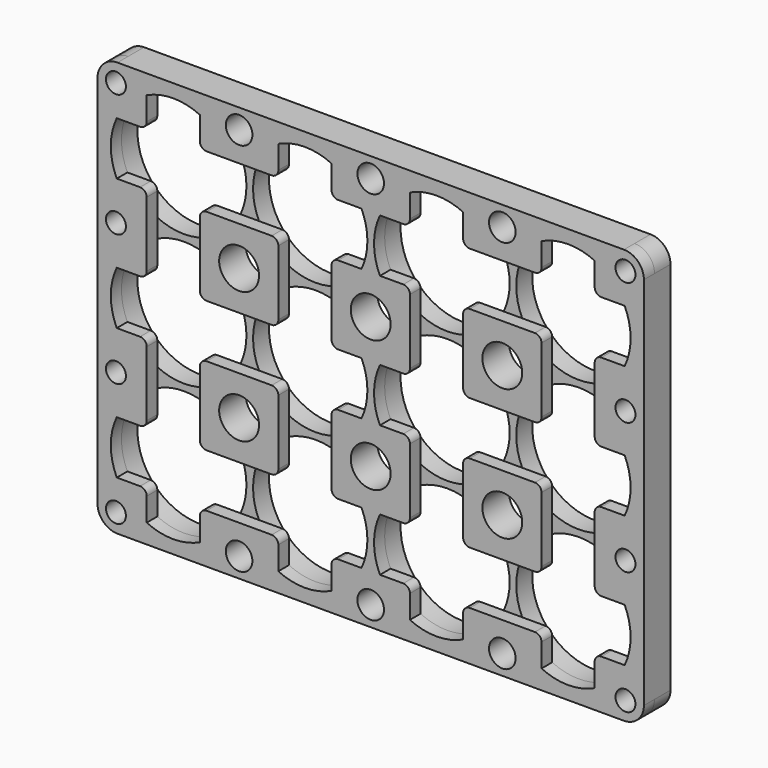
from build123d import *

# Parameters (mm, degrees)
F0_W     = 82.2
F0_H     = 62.4
F0_R     = 1.5
F0_R_2   = 9.4
F0_R_3   = 2
F0_R_4   = 3
F1_DEPTH = 3
F2_R     = 3
F3_R     = 1.5
F3_R_2   = 2
F3_R_3   = 3
F4_DEPTH = 2
F5_R     = 1


# Not quite as in the source:
# - after a boolean that leaves OpenCascade's solid faulty, fix() repairs it


with BuildPart() as f1:
    # F0 (on Front) → F1 (new body)
    with BuildSketch(Plane.XZ):
        with Locations((29.7, 19.8)):
            Rectangle(F0_W, F0_H)
        with Locations((-8.630645927, -8.630645927)):
            Circle(F0_R, mode=Mode.SUBTRACT)
        Circle(F0_R_2, mode=Mode.SUBTRACT)
        with Locations((9.9, -8.4255563615)):
            Circle(F0_R_3, mode=Mode.SUBTRACT)
        with Locations((19.8, 0)):
            Circle(F0_R_2, mode=Mode.SUBTRACT)
        with Locations((-8.630645927, 9.9)):
            Circle(F0_R, mode=Mode.SUBTRACT)
        with Locations((9.9, 9.9)):
            Circle(F0_R_4, mode=Mode.SUBTRACT)
        with Locations((29.7, -8.4255563615)):
            Circle(F0_R_3, mode=Mode.SUBTRACT)
        with Locations((49.5, -8.4255563615)):
            Circle(F0_R_3, mode=Mode.SUBTRACT)
        with Locations((39.6, 0)):
            Circle(F0_R_2, mode=Mode.SUBTRACT)
        with Locations((68.030645927, -8.630645927)):
            Circle(F0_R, mode=Mode.SUBTRACT)
        with Locations((59.4, 0)):
            Circle(F0_R_2, mode=Mode.SUBTRACT)
        with Locations((29.7, 9.9)):
            Circle(F0_R_4, mode=Mode.SUBTRACT)
        with Locations((49.5, 9.9)):
            Circle(F0_R_4, mode=Mode.SUBTRACT)
        with Locations((68.030645927, 9.9)):
            Circle(F0_R, mode=Mode.SUBTRACT)
        with Locations((0, 19.8)):
            Circle(F0_R_2, mode=Mode.SUBTRACT)
        with Locations((-8.630645927, 29.7)):
            Circle(F0_R, mode=Mode.SUBTRACT)
        with Locations((19.8, 19.8)):
            Circle(F0_R_2, mode=Mode.SUBTRACT)
        with Locations((9.9, 29.7)):
            Circle(F0_R_4, mode=Mode.SUBTRACT)
        with Locations((0, 39.6)):
            Circle(F0_R_2, mode=Mode.SUBTRACT)
        with Locations((-8.630645927, 48.230645927)):
            Circle(F0_R, mode=Mode.SUBTRACT)
        with Locations((19.8, 39.6)):
            Circle(F0_R_2, mode=Mode.SUBTRACT)
        with Locations((9.9, 48.0255563615)):
            Circle(F0_R_3, mode=Mode.SUBTRACT)
        with Locations((39.6, 19.8)):
            Circle(F0_R_2, mode=Mode.SUBTRACT)
        with Locations((29.7, 29.7)):
            Circle(F0_R_4, mode=Mode.SUBTRACT)
        with Locations((49.5, 29.7)):
            Circle(F0_R_4, mode=Mode.SUBTRACT)
        with Locations((59.4, 19.8)):
            Circle(F0_R_2, mode=Mode.SUBTRACT)
        with Locations((68.030645927, 29.7)):
            Circle(F0_R, mode=Mode.SUBTRACT)
        with Locations((39.6, 39.6)):
            Circle(F0_R_2, mode=Mode.SUBTRACT)
        with Locations((29.7, 48.0255563615)):
            Circle(F0_R_3, mode=Mode.SUBTRACT)
        with Locations((49.5, 48.0255563615)):
            Circle(F0_R_3, mode=Mode.SUBTRACT)
        with Locations((59.4, 39.6)):
            Circle(F0_R_2, mode=Mode.SUBTRACT)
        with Locations((68.030645927, 48.230645927)):
            Circle(F0_R, mode=Mode.SUBTRACT)
    extrude(amount=F1_DEPTH)

    # F2
    f2_edges = [f1.edges().sort_by_distance(p)[0] for p in [
        (70.8, -1.5, 51),
        (-11.4, -1.5, 51),
        (-11.4, -1.5, -11.4),
        (70.8, -1.5, -11.4),
    ]]
    fillet(f2_edges, radius=F2_R)

    # F3 (on face) → F4 (join)
    with BuildSketch(Plane.XZ.offset(3)):
        with BuildLine():
            ThreePointArc((70.8, 48), (69.9213203436, 50.1213203436), (67.8, 51))
            Line((67.8, 51), (63.4, 51))
            Line((63.4, 51), (63.4, 48.1064681273))
            ThreePointArc((63.4, 48.1064681273), (66.0468037432, 46.2468037432), (67.9064681273, 43.6))
            Line((67.9064681273, 43.6), (70.8, 43.6))
            Line((70.8, 43.6), (70.8, 48))
        make_face()
        with Locations((68.030645927, 48.230645927)):
            Circle(F3_R, mode=Mode.SUBTRACT)
        with BuildLine():
            Line((63.4, 48.1064681273), (63.4, 51))
            Line((63.4, 51), (55.4, 51))
            Line((55.4, 51), (55.4, 48.1064681273))
            ThreePointArc((55.4, 48.1064681273), (59.4, 49), (63.4, 48.1064681273))
        make_face()
        with BuildLine():
            Line((55.4, 48.1064681273), (55.4, 51))
            Line((55.4, 51), (43.6, 51))
            Line((43.6, 51), (43.6, 48.1064681273))
            ThreePointArc((43.6, 48.1064681273), (46.2468037432, 46.2468037432), (48.1064681273, 43.6))
            Line((48.1064681273, 43.6), (50.8935318727, 43.6))
            ThreePointArc((50.8935318727, 43.6), (52.7531962568, 46.2468037432), (55.4, 48.1064681273))
        make_face()
        with Locations((49.5, 48.0255563615)):
            Circle(F3_R_2, mode=Mode.SUBTRACT)
        with BuildLine():
            ThreePointArc((67.9064681273, 43.6), (66.0468037432, 46.2468037432), (63.4, 48.1064681273))
            Line((63.4, 48.1064681273), (63.4, 43.6))
            Line((63.4, 43.6), (67.9064681273, 43.6))
        make_face()
        with BuildLine():
            Line((70.8, 39.6), (70.8, 43.6))
            Line((70.8, 43.6), (67.9064681273, 43.6))
            ThreePointArc((67.9064681273, 43.6), (68.5738977648, 41.6492925125), (68.8, 39.6))
            ThreePointArc((68.8, 39.6), (68.5738977648, 37.5507074875), (67.9064681273, 35.6))
            Line((67.9064681273, 35.6), (70.8, 35.6))
            Line((70.8, 35.6), (70.8, 39.6))
        make_face()
        with BuildLine():
            Line((43.6, 48.1064681273), (43.6, 51))
            Line((43.6, 51), (35.6, 51))
            Line((35.6, 51), (35.6, 48.1064681273))
            ThreePointArc((35.6, 48.1064681273), (39.6, 49), (43.6, 48.1064681273))
        make_face()
        with BuildLine():
            Line((55.4, 43.6), (55.4, 48.1064681273))
            ThreePointArc((55.4, 48.1064681273), (52.7531962568, 46.2468037432), (50.8935318727, 43.6))
            Line((50.8935318727, 43.6), (55.4, 43.6))
        make_face()
        with BuildLine():
            Line((35.6, 48.1064681273), (35.6, 51))
            Line((35.6, 51), (23.8, 51))
            Line((23.8, 51), (23.8, 48.1064681273))
            ThreePointArc((23.8, 48.1064681273), (26.4468037432, 46.2468037432), (28.3064681273, 43.6))
            Line((28.3064681273, 43.6), (31.0935318727, 43.6))
            ThreePointArc((31.0935318727, 43.6), (32.9531962568, 46.2468037432), (35.6, 48.1064681273))
        make_face()
        with Locations((29.7, 48.0255563615)):
            Circle(F3_R_2, mode=Mode.SUBTRACT)
        with BuildLine():
            ThreePointArc((48.1064681273, 43.6), (46.2468037432, 46.2468037432), (43.6, 48.1064681273))
            Line((43.6, 48.1064681273), (43.6, 43.6))
            Line((43.6, 43.6), (48.1064681273, 43.6))
        make_face()
        with BuildLine():
            Line((70.8, 23.8), (70.8, 35.6))
            Line((70.8, 35.6), (67.9064681273, 35.6))
            ThreePointArc((67.9064681273, 35.6), (66.0468037432, 32.9531962568), (63.4, 31.0935318727))
            Line((63.4, 31.0935318727), (63.4, 28.3064681273))
            ThreePointArc((63.4, 28.3064681273), (66.0468037432, 26.4468037432), (67.9064681273, 23.8))
            Line((67.9064681273, 23.8), (70.8, 23.8))
        make_face()
        with Locations((68.030645927, 29.7)):
            Circle(F3_R, mode=Mode.SUBTRACT)
        with BuildLine():
            Line((23.8, 48.1064681273), (23.8, 51))
            Line((23.8, 51), (15.8, 51))
            Line((15.8, 51), (15.8, 48.1064681273))
            ThreePointArc((15.8, 48.1064681273), (19.8, 49), (23.8, 48.1064681273))
        make_face()
        with BuildLine():
            Line((35.6, 43.6), (35.6, 48.1064681273))
            ThreePointArc((35.6, 48.1064681273), (32.9531962568, 46.2468037432), (31.0935318727, 43.6))
            Line((31.0935318727, 43.6), (35.6, 43.6))
        make_face()
        with BuildLine():
            Line((55.4, 35.6), (50.8935318727, 35.6))
            ThreePointArc((50.8935318727, 35.6), (52.7531962568, 32.9531962568), (55.4, 31.0935318727))
            Line((55.4, 31.0935318727), (55.4, 35.6))
        make_face()
        with BuildLine():
            ThreePointArc((55.4, 31.0935318727), (52.7531962568, 32.9531962568), (50.8935318727, 35.6))
            Line((50.8935318727, 35.6), (48.1064681273, 35.6))
            ThreePointArc((48.1064681273, 35.6), (46.2468037432, 32.9531962568), (43.6, 31.0935318727))
            Line((43.6, 31.0935318727), (43.6, 28.3064681273))
            ThreePointArc((43.6, 28.3064681273), (46.2468037432, 26.4468037432), (48.1064681273, 23.8))
            Line((48.1064681273, 23.8), (50.8935318727, 23.8))
            ThreePointArc((50.8935318727, 23.8), (52.7531962568, 26.4468037432), (55.4, 28.3064681273))
            Line((55.4, 28.3064681273), (55.4, 31.0935318727))
        make_face()
        with Locations((49.5, 29.7)):
            Circle(F3_R_3, mode=Mode.SUBTRACT)
        with BuildLine():
            ThreePointArc((63.4, 31.0935318727), (66.0468037432, 32.9531962568), (67.9064681273, 35.6))
            Line((67.9064681273, 35.6), (63.4, 35.6))
            Line((63.4, 35.6), (63.4, 31.0935318727))
        make_face()
        with BuildLine():
            Line((70.8, 15.8), (70.8, 23.8))
            Line((70.8, 23.8), (67.9064681273, 23.8))
            ThreePointArc((67.9064681273, 23.8), (68.5738977648, 21.8492925125), (68.8, 19.8))
            ThreePointArc((68.8, 19.8), (68.5738977648, 17.7507074875), (67.9064681273, 15.8))
            Line((67.9064681273, 15.8), (70.8, 15.8))
        make_face()
        with BuildLine():
            Line((15.8, 48.1064681273), (15.8, 51))
            Line((15.8, 51), (4, 51))
            Line((4, 51), (4, 48.1064681273))
            ThreePointArc((4, 48.1064681273), (6.6468037432, 46.2468037432), (8.5064681273, 43.6))
            Line((8.5064681273, 43.6), (11.2935318727, 43.6))
            ThreePointArc((11.2935318727, 43.6), (13.1531962568, 46.2468037432), (15.8, 48.1064681273))
        make_face()
        with Locations((9.9, 48.0255563615)):
            Circle(F3_R_2, mode=Mode.SUBTRACT)
        with BuildLine():
            ThreePointArc((28.3064681273, 43.6), (26.4468037432, 46.2468037432), (23.8, 48.1064681273))
            Line((23.8, 48.1064681273), (23.8, 43.6))
            Line((23.8, 43.6), (28.3064681273, 43.6))
        make_face()
        with BuildLine():
            ThreePointArc((31.0935318727, 35.6), (30.2, 39.6), (31.0935318727, 43.6))
            Line((31.0935318727, 43.6), (28.3064681273, 43.6))
            ThreePointArc((28.3064681273, 43.6), (28.9738977648, 41.6492925125), (29.2, 39.6))
            ThreePointArc((29.2, 39.6), (28.9738977648, 37.5507074875), (28.3064681273, 35.6))
            Line((28.3064681273, 35.6), (31.0935318727, 35.6))
        make_face()
        with BuildLine():
            ThreePointArc((43.6, 31.0935318727), (46.2468037432, 32.9531962568), (48.1064681273, 35.6))
            Line((48.1064681273, 35.6), (43.6, 35.6))
            Line((43.6, 35.6), (43.6, 31.0935318727))
        make_face()
        with BuildLine():
            Line((70.8, 4), (70.8, 15.8))
            Line((70.8, 15.8), (67.9064681273, 15.8))
            ThreePointArc((67.9064681273, 15.8), (66.0468037432, 13.1531962568), (63.4, 11.2935318727))
            Line((63.4, 11.2935318727), (63.4, 8.5064681273))
            ThreePointArc((63.4, 8.5064681273), (66.0468037432, 6.6468037432), (67.9064681273, 4))
            Line((67.9064681273, 4), (70.8, 4))
        make_face()
        with Locations((68.030645927, 9.9)):
            Circle(F3_R, mode=Mode.SUBTRACT)
        with BuildLine():
            Line((63.4, 23.8), (67.9064681273, 23.8))
            ThreePointArc((67.9064681273, 23.8), (66.0468037432, 26.4468037432), (63.4, 28.3064681273))
            Line((63.4, 28.3064681273), (63.4, 23.8))
        make_face()
        with BuildLine():
            Line((4, 48.1064681273), (4, 51))
            Line((4, 51), (-4, 51))
            Line((-4, 51), (-4, 48.1064681273))
            ThreePointArc((-4, 48.1064681273), (0, 49), (4, 48.1064681273))
        make_face()
        with BuildLine():
            Line((15.8, 43.6), (15.8, 48.1064681273))
            ThreePointArc((15.8, 48.1064681273), (13.1531962568, 46.2468037432), (11.2935318727, 43.6))
            Line((11.2935318727, 43.6), (15.8, 43.6))
        make_face()
        with BuildLine():
            Line((35.6, 35.6), (31.0935318727, 35.6))
            ThreePointArc((31.0935318727, 35.6), (32.9531962568, 32.9531962568), (35.6, 31.0935318727))
            Line((35.6, 31.0935318727), (35.6, 35.6))
        make_face()
        with BuildLine():
            ThreePointArc((35.6, 31.0935318727), (32.9531962568, 32.9531962568), (31.0935318727, 35.6))
            Line((31.0935318727, 35.6), (28.3064681273, 35.6))
            ThreePointArc((28.3064681273, 35.6), (26.4468037432, 32.9531962568), (23.8, 31.0935318727))
            Line((23.8, 31.0935318727), (23.8, 28.3064681273))
            ThreePointArc((23.8, 28.3064681273), (26.4468037432, 26.4468037432), (28.3064681273, 23.8))
            Line((28.3064681273, 23.8), (31.0935318727, 23.8))
            ThreePointArc((31.0935318727, 23.8), (32.9531962568, 26.4468037432), (35.6, 28.3064681273))
            Line((35.6, 28.3064681273), (35.6, 31.0935318727))
        make_face()
        with Locations((29.7, 29.7)):
            Circle(F3_R_3, mode=Mode.SUBTRACT)
        with BuildLine():
            Line((55.4, 23.8), (55.4, 28.3064681273))
            ThreePointArc((55.4, 28.3064681273), (52.7531962568, 26.4468037432), (50.8935318727, 23.8))
            Line((50.8935318727, 23.8), (55.4, 23.8))
        make_face()
        with BuildLine():
            Line((70.8, -4), (70.8, 4))
            Line((70.8, 4), (67.9064681273, 4))
            ThreePointArc((67.9064681273, 4), (68.5738977648, 2.0492925125), (68.8, 0))
            ThreePointArc((68.8, 0), (68.5738977648, -2.0492925125), (67.9064681273, -4))
            Line((67.9064681273, -4), (70.8, -4))
        make_face()
        with BuildLine():
            ThreePointArc((63.4, 11.2935318727), (66.0468037432, 13.1531962568), (67.9064681273, 15.8))
            Line((67.9064681273, 15.8), (63.4, 15.8))
            Line((63.4, 15.8), (63.4, 11.2935318727))
        make_face()
        with BuildLine():
            Line((-4, 48.1064681273), (-4, 51))
            Line((-4, 51), (-8.4, 51))
            ThreePointArc((-8.4, 51), (-10.5213203436, 50.1213203436), (-11.4, 48))
            Line((-11.4, 48), (-11.4, 43.6))
            Line((-11.4, 43.6), (-8.5064681273, 43.6))
            ThreePointArc((-8.5064681273, 43.6), (-6.6468037432, 46.2468037432), (-4, 48.1064681273))
        make_face()
        with Locations((-8.630645927, 48.230645927)):
            Circle(F3_R, mode=Mode.SUBTRACT)
        with BuildLine():
            ThreePointArc((8.5064681273, 43.6), (6.6468037432, 46.2468037432), (4, 48.1064681273))
            Line((4, 48.1064681273), (4, 43.6))
            Line((4, 43.6), (8.5064681273, 43.6))
        make_face()
        with BuildLine():
            ThreePointArc((23.8, 31.0935318727), (26.4468037432, 32.9531962568), (28.3064681273, 35.6))
            Line((28.3064681273, 35.6), (23.8, 35.6))
            Line((23.8, 35.6), (23.8, 31.0935318727))
        make_face()
        with BuildLine():
            ThreePointArc((48.1064681273, 23.8), (46.2468037432, 26.4468037432), (43.6, 28.3064681273))
            Line((43.6, 28.3064681273), (43.6, 23.8))
            Line((43.6, 23.8), (48.1064681273, 23.8))
        make_face()
        with BuildLine():
            Line((70.8, -8.4), (70.8, -4))
            Line((70.8, -4), (67.9064681273, -4))
            ThreePointArc((67.9064681273, -4), (66.0468037432, -6.6468037432), (63.4, -8.5064681273))
            Line((63.4, -8.5064681273), (63.4, -11.4))
            Line((63.4, -11.4), (67.8, -11.4))
            ThreePointArc((67.8, -11.4), (69.9213203436, -10.5213203436), (70.8, -8.4))
        make_face()
        with Locations((68.030645927, -8.630645927)):
            Circle(F3_R, mode=Mode.SUBTRACT)
        with BuildLine():
            Line((63.4, 4), (67.9064681273, 4))
            ThreePointArc((67.9064681273, 4), (66.0468037432, 6.6468037432), (63.4, 8.5064681273))
            Line((63.4, 8.5064681273), (63.4, 4))
        make_face()
        with BuildLine():
            Line((-4, 43.6), (-4, 48.1064681273))
            ThreePointArc((-4, 48.1064681273), (-6.6468037432, 46.2468037432), (-8.5064681273, 43.6))
            Line((-8.5064681273, 43.6), (-4, 43.6))
        make_face()
        with BuildLine():
            Line((15.8, 35.6), (11.2935318727, 35.6))
            ThreePointArc((11.2935318727, 35.6), (13.1531962568, 32.9531962568), (15.8, 31.0935318727))
            Line((15.8, 31.0935318727), (15.8, 35.6))
        make_face()
        with BuildLine():
            ThreePointArc((15.8, 31.0935318727), (13.1531962568, 32.9531962568), (11.2935318727, 35.6))
            Line((11.2935318727, 35.6), (8.5064681273, 35.6))
            ThreePointArc((8.5064681273, 35.6), (6.6468037432, 32.9531962568), (4, 31.0935318727))
            Line((4, 31.0935318727), (4, 28.3064681273))
            ThreePointArc((4, 28.3064681273), (6.6468037432, 26.4468037432), (8.5064681273, 23.8))
            Line((8.5064681273, 23.8), (11.2935318727, 23.8))
            ThreePointArc((11.2935318727, 23.8), (13.1531962568, 26.4468037432), (15.8, 28.3064681273))
            Line((15.8, 28.3064681273), (15.8, 31.0935318727))
        make_face()
        with Locations((9.9, 29.7)):
            Circle(F3_R_3, mode=Mode.SUBTRACT)
        with BuildLine():
            Line((35.6, 23.8), (35.6, 28.3064681273))
            ThreePointArc((35.6, 28.3064681273), (32.9531962568, 26.4468037432), (31.0935318727, 23.8))
            Line((31.0935318727, 23.8), (35.6, 23.8))
        make_face()
        with BuildLine():
            Line((55.4, 15.8), (50.8935318727, 15.8))
            ThreePointArc((50.8935318727, 15.8), (52.7531962568, 13.1531962568), (55.4, 11.2935318727))
            Line((55.4, 11.2935318727), (55.4, 15.8))
        make_face()
        with BuildLine():
            ThreePointArc((55.4, 11.2935318727), (52.7531962568, 13.1531962568), (50.8935318727, 15.8))
            Line((50.8935318727, 15.8), (48.1064681273, 15.8))
            ThreePointArc((48.1064681273, 15.8), (46.2468037432, 13.1531962568), (43.6, 11.2935318727))
            Line((43.6, 11.2935318727), (43.6, 8.5064681273))
            ThreePointArc((43.6, 8.5064681273), (46.2468037432, 6.6468037432), (48.1064681273, 4))
            Line((48.1064681273, 4), (50.8935318727, 4))
            ThreePointArc((50.8935318727, 4), (52.7531962568, 6.6468037432), (55.4, 8.5064681273))
            Line((55.4, 8.5064681273), (55.4, 11.2935318727))
        make_face()
        with Locations((49.5, 9.9)):
            Circle(F3_R_3, mode=Mode.SUBTRACT)
        with BuildLine():
            ThreePointArc((63.4, -8.5064681273), (66.0468037432, -6.6468037432), (67.9064681273, -4))
            Line((67.9064681273, -4), (63.4, -4))
            Line((63.4, -4), (63.4, -8.5064681273))
        make_face()
        with BuildLine():
            ThreePointArc((-8.5064681273, 35.6), (-9.4, 39.6), (-8.5064681273, 43.6))
            Line((-8.5064681273, 43.6), (-11.4, 43.6))
            Line((-11.4, 43.6), (-11.4, 39.6))
            Line((-11.4, 39.6), (-11.4, 35.6))
            Line((-11.4, 35.6), (-8.5064681273, 35.6))
        make_face()
        with BuildLine():
            ThreePointArc((4, 31.0935318727), (6.6468037432, 32.9531962568), (8.5064681273, 35.6))
            Line((8.5064681273, 35.6), (4, 35.6))
            Line((4, 35.6), (4, 31.0935318727))
        make_face()
        with BuildLine():
            ThreePointArc((31.0935318727, 15.8), (30.2, 19.8), (31.0935318727, 23.8))
            Line((31.0935318727, 23.8), (28.3064681273, 23.8))
            ThreePointArc((28.3064681273, 23.8), (28.9738977648, 21.8492925125), (29.2, 19.8))
            ThreePointArc((29.2, 19.8), (28.9738977648, 17.7507074875), (28.3064681273, 15.8))
            Line((28.3064681273, 15.8), (31.0935318727, 15.8))
        make_face()
        with BuildLine():
            ThreePointArc((28.3064681273, 23.8), (26.4468037432, 26.4468037432), (23.8, 28.3064681273))
            Line((23.8, 28.3064681273), (23.8, 23.8))
            Line((23.8, 23.8), (28.3064681273, 23.8))
        make_face()
        with BuildLine():
            ThreePointArc((43.6, 11.2935318727), (46.2468037432, 13.1531962568), (48.1064681273, 15.8))
            Line((48.1064681273, 15.8), (43.6, 15.8))
            Line((43.6, 15.8), (43.6, 11.2935318727))
        make_face()
        with BuildLine():
            Line((63.4, -11.4), (63.4, -8.5064681273))
            ThreePointArc((63.4, -8.5064681273), (59.4, -9.4), (55.4, -8.5064681273))
            Line((55.4, -8.5064681273), (55.4, -11.4))
            Line((55.4, -11.4), (63.4, -11.4))
        make_face()
        with BuildLine():
            Line((55.4, 4), (55.4, 8.5064681273))
            ThreePointArc((55.4, 8.5064681273), (52.7531962568, 6.6468037432), (50.8935318727, 4))
            Line((50.8935318727, 4), (55.4, 4))
        make_face()
        with BuildLine():
            ThreePointArc((-4, 31.0935318727), (-6.6468037432, 32.9531962568), (-8.5064681273, 35.6))
            Line((-8.5064681273, 35.6), (-11.4, 35.6))
            Line((-11.4, 35.6), (-11.4, 23.8))
            Line((-11.4, 23.8), (-8.5064681273, 23.8))
            ThreePointArc((-8.5064681273, 23.8), (-6.6468037432, 26.4468037432), (-4, 28.3064681273))
            Line((-4, 28.3064681273), (-4, 31.0935318727))
        make_face()
        with Locations((-8.630645927, 29.7)):
            Circle(F3_R, mode=Mode.SUBTRACT)
        with BuildLine():
            Line((-4, 35.6), (-8.5064681273, 35.6))
            ThreePointArc((-8.5064681273, 35.6), (-6.6468037432, 32.9531962568), (-4, 31.0935318727))
            Line((-4, 31.0935318727), (-4, 35.6))
        make_face()
        with BuildLine():
            Line((15.8, 23.8), (15.8, 28.3064681273))
            ThreePointArc((15.8, 28.3064681273), (13.1531962568, 26.4468037432), (11.2935318727, 23.8))
            Line((11.2935318727, 23.8), (15.8, 23.8))
        make_face()
        with BuildLine():
            Line((35.6, 15.8), (31.0935318727, 15.8))
            ThreePointArc((31.0935318727, 15.8), (32.9531962568, 13.1531962568), (35.6, 11.2935318727))
            Line((35.6, 11.2935318727), (35.6, 15.8))
        make_face()
        with BuildLine():
            ThreePointArc((35.6, 11.2935318727), (32.9531962568, 13.1531962568), (31.0935318727, 15.8))
            Line((31.0935318727, 15.8), (28.3064681273, 15.8))
            ThreePointArc((28.3064681273, 15.8), (26.4468037432, 13.1531962568), (23.8, 11.2935318727))
            Line((23.8, 11.2935318727), (23.8, 8.5064681273))
            ThreePointArc((23.8, 8.5064681273), (26.4468037432, 6.6468037432), (28.3064681273, 4))
            Line((28.3064681273, 4), (31.0935318727, 4))
            ThreePointArc((31.0935318727, 4), (32.9531962568, 6.6468037432), (35.6, 8.5064681273))
            Line((35.6, 8.5064681273), (35.6, 11.2935318727))
        make_face()
        with Locations((29.7, 9.9)):
            Circle(F3_R_3, mode=Mode.SUBTRACT)
        with BuildLine():
            Line((55.4, -11.4), (55.4, -8.5064681273))
            ThreePointArc((55.4, -8.5064681273), (52.7531962568, -6.6468037432), (50.8935318727, -4))
            Line((50.8935318727, -4), (48.1064681273, -4))
            ThreePointArc((48.1064681273, -4), (46.2468037432, -6.6468037432), (43.6, -8.5064681273))
            Line((43.6, -8.5064681273), (43.6, -11.4))
            Line((43.6, -11.4), (55.4, -11.4))
        make_face()
        with Locations((49.5, -8.4255563615)):
            Circle(F3_R_2, mode=Mode.SUBTRACT)
        with BuildLine():
            ThreePointArc((50.8935318727, -4), (52.7531962568, -6.6468037432), (55.4, -8.5064681273))
            Line((55.4, -8.5064681273), (55.4, -4))
            Line((55.4, -4), (50.8935318727, -4))
        make_face()
        with BuildLine():
            ThreePointArc((8.5064681273, 23.8), (6.6468037432, 26.4468037432), (4, 28.3064681273))
            Line((4, 28.3064681273), (4, 23.8))
            Line((4, 23.8), (8.5064681273, 23.8))
        make_face()
        with BuildLine():
            ThreePointArc((23.8, 11.2935318727), (26.4468037432, 13.1531962568), (28.3064681273, 15.8))
            Line((28.3064681273, 15.8), (23.8, 15.8))
            Line((23.8, 15.8), (23.8, 11.2935318727))
        make_face()
        with BuildLine():
            ThreePointArc((48.1064681273, 4), (46.2468037432, 6.6468037432), (43.6, 8.5064681273))
            Line((43.6, 8.5064681273), (43.6, 4))
            Line((43.6, 4), (48.1064681273, 4))
        make_face()
        with BuildLine():
            Line((-8.5064681273, 23.8), (-11.4, 23.8))
            Line((-11.4, 23.8), (-11.4, 15.8))
            Line((-11.4, 15.8), (-8.5064681273, 15.8))
            ThreePointArc((-8.5064681273, 15.8), (-9.4, 19.8), (-8.5064681273, 23.8))
        make_face()
        with BuildLine():
            Line((-4, 23.8), (-4, 28.3064681273))
            ThreePointArc((-4, 28.3064681273), (-6.6468037432, 26.4468037432), (-8.5064681273, 23.8))
            Line((-8.5064681273, 23.8), (-4, 23.8))
        make_face()
        with BuildLine():
            Line((15.8, 15.8), (11.2935318727, 15.8))
            ThreePointArc((11.2935318727, 15.8), (13.1531962568, 13.1531962568), (15.8, 11.2935318727))
            Line((15.8, 11.2935318727), (15.8, 15.8))
        make_face()
        with BuildLine():
            ThreePointArc((15.8, 11.2935318727), (13.1531962568, 13.1531962568), (11.2935318727, 15.8))
            Line((11.2935318727, 15.8), (8.5064681273, 15.8))
            ThreePointArc((8.5064681273, 15.8), (6.6468037432, 13.1531962568), (4, 11.2935318727))
            Line((4, 11.2935318727), (4, 8.5064681273))
            ThreePointArc((4, 8.5064681273), (6.6468037432, 6.6468037432), (8.5064681273, 4))
            Line((8.5064681273, 4), (11.2935318727, 4))
            ThreePointArc((11.2935318727, 4), (13.1531962568, 6.6468037432), (15.8, 8.5064681273))
            Line((15.8, 8.5064681273), (15.8, 11.2935318727))
        make_face()
        with Locations((9.9, 9.9)):
            Circle(F3_R_3, mode=Mode.SUBTRACT)
        with BuildLine():
            Line((35.6, 4), (35.6, 8.5064681273))
            ThreePointArc((35.6, 8.5064681273), (32.9531962568, 6.6468037432), (31.0935318727, 4))
            Line((31.0935318727, 4), (35.6, 4))
        make_face()
        with BuildLine():
            Line((35.6, -11.4), (43.6, -11.4))
            Line((43.6, -11.4), (43.6, -8.5064681273))
            ThreePointArc((43.6, -8.5064681273), (39.6, -9.4), (35.6, -8.5064681273))
            Line((35.6, -8.5064681273), (35.6, -11.4))
        make_face()
        with BuildLine():
            ThreePointArc((43.6, -8.5064681273), (46.2468037432, -6.6468037432), (48.1064681273, -4))
            Line((48.1064681273, -4), (43.6, -4))
            Line((43.6, -4), (43.6, -8.5064681273))
        make_face()
        with BuildLine():
            Line((-8.5064681273, 15.8), (-11.4, 15.8))
            Line((-11.4, 15.8), (-11.4, 4))
            Line((-11.4, 4), (-8.5064681273, 4))
            ThreePointArc((-8.5064681273, 4), (-6.6468037432, 6.6468037432), (-4, 8.5064681273))
            Line((-4, 8.5064681273), (-4, 11.2935318727))
            ThreePointArc((-4, 11.2935318727), (-6.6468037432, 13.1531962568), (-8.5064681273, 15.8))
        make_face()
        with Locations((-8.630645927, 9.9)):
            Circle(F3_R, mode=Mode.SUBTRACT)
        with BuildLine():
            ThreePointArc((4, 11.2935318727), (6.6468037432, 13.1531962568), (8.5064681273, 15.8))
            Line((8.5064681273, 15.8), (4, 15.8))
            Line((4, 15.8), (4, 11.2935318727))
        make_face()
        with BuildLine():
            ThreePointArc((31.0935318727, -4), (30.2, 0), (31.0935318727, 4))
            Line((31.0935318727, 4), (28.3064681273, 4))
            ThreePointArc((28.3064681273, 4), (28.9738977648, 2.0492925125), (29.2, 0))
            ThreePointArc((29.2, 0), (28.9738977648, -2.0492925125), (28.3064681273, -4))
            Line((28.3064681273, -4), (31.0935318727, -4))
        make_face()
        with BuildLine():
            ThreePointArc((28.3064681273, 4), (26.4468037432, 6.6468037432), (23.8, 8.5064681273))
            Line((23.8, 8.5064681273), (23.8, 4))
            Line((23.8, 4), (28.3064681273, 4))
        make_face()
        with BuildLine():
            Line((23.8, -11.4), (35.6, -11.4))
            Line((35.6, -11.4), (35.6, -8.5064681273))
            ThreePointArc((35.6, -8.5064681273), (32.9531962568, -6.6468037432), (31.0935318727, -4))
            Line((31.0935318727, -4), (28.3064681273, -4))
            ThreePointArc((28.3064681273, -4), (26.4468037432, -6.6468037432), (23.8, -8.5064681273))
            Line((23.8, -8.5064681273), (23.8, -11.4))
        make_face()
        with Locations((29.7, -8.4255563615)):
            Circle(F3_R_2, mode=Mode.SUBTRACT)
        with BuildLine():
            Line((-8.5064681273, 4), (-11.4, 4))
            Line((-11.4, 4), (-11.4, -4))
            Line((-11.4, -4), (-8.5064681273, -4))
            ThreePointArc((-8.5064681273, -4), (-9.4, 0), (-8.5064681273, 4))
        make_face()
        with BuildLine():
            Line((-4, 15.8), (-8.5064681273, 15.8))
            ThreePointArc((-8.5064681273, 15.8), (-6.6468037432, 13.1531962568), (-4, 11.2935318727))
            Line((-4, 11.2935318727), (-4, 15.8))
        make_face()
        with BuildLine():
            Line((15.8, 4), (15.8, 8.5064681273))
            ThreePointArc((15.8, 8.5064681273), (13.1531962568, 6.6468037432), (11.2935318727, 4))
            Line((11.2935318727, 4), (15.8, 4))
        make_face()
        with BuildLine():
            Line((35.6, -4), (31.0935318727, -4))
            ThreePointArc((31.0935318727, -4), (32.9531962568, -6.6468037432), (35.6, -8.5064681273))
            Line((35.6, -8.5064681273), (35.6, -4))
        make_face()
        with BuildLine():
            Line((15.8, -11.4), (23.8, -11.4))
            Line((23.8, -11.4), (23.8, -8.5064681273))
            ThreePointArc((23.8, -8.5064681273), (19.8, -9.4), (15.8, -8.5064681273))
            Line((15.8, -8.5064681273), (15.8, -11.4))
        make_face()
        with BuildLine():
            Line((-8.5064681273, -4), (-11.4, -4))
            Line((-11.4, -4), (-11.4, -8.4))
            ThreePointArc((-11.4, -8.4), (-10.5213203436, -10.5213203436), (-8.4, -11.4))
            Line((-8.4, -11.4), (-4, -11.4))
            Line((-4, -11.4), (-4, -8.5064681273))
            ThreePointArc((-4, -8.5064681273), (-6.6468037432, -6.6468037432), (-8.5064681273, -4))
        make_face()
        with Locations((-8.630645927, -8.630645927)):
            Circle(F3_R, mode=Mode.SUBTRACT)
        with BuildLine():
            ThreePointArc((-4, 8.5064681273), (-6.6468037432, 6.6468037432), (-8.5064681273, 4))
            Line((-8.5064681273, 4), (-4, 4))
            Line((-4, 4), (-4, 8.5064681273))
        make_face()
        with BuildLine():
            ThreePointArc((8.5064681273, 4), (6.6468037432, 6.6468037432), (4, 8.5064681273))
            Line((4, 8.5064681273), (4, 4))
            Line((4, 4), (8.5064681273, 4))
        make_face()
        with BuildLine():
            ThreePointArc((23.8, -8.5064681273), (26.4468037432, -6.6468037432), (28.3064681273, -4))
            Line((28.3064681273, -4), (23.8, -4))
            Line((23.8, -4), (23.8, -8.5064681273))
        make_face()
        with BuildLine():
            Line((4, -11.4), (15.8, -11.4))
            Line((15.8, -11.4), (15.8, -8.5064681273))
            ThreePointArc((15.8, -8.5064681273), (13.1531962568, -6.6468037432), (11.2935318727, -4))
            Line((11.2935318727, -4), (8.5064681273, -4))
            ThreePointArc((8.5064681273, -4), (6.6468037432, -6.6468037432), (4, -8.5064681273))
            Line((4, -8.5064681273), (4, -11.4))
        make_face()
        with Locations((9.9, -8.4255563615)):
            Circle(F3_R_2, mode=Mode.SUBTRACT)
        with BuildLine():
            Line((-4, -4), (-8.5064681273, -4))
            ThreePointArc((-8.5064681273, -4), (-6.6468037432, -6.6468037432), (-4, -8.5064681273))
            Line((-4, -8.5064681273), (-4, -4))
        make_face()
        with BuildLine():
            Line((15.8, -4), (11.2935318727, -4))
            ThreePointArc((11.2935318727, -4), (13.1531962568, -6.6468037432), (15.8, -8.5064681273))
            Line((15.8, -8.5064681273), (15.8, -4))
        make_face()
        with BuildLine():
            Line((-4, -11.4), (4, -11.4))
            Line((4, -11.4), (4, -8.5064681273))
            ThreePointArc((4, -8.5064681273), (0, -9.4), (-4, -8.5064681273))
            Line((-4, -8.5064681273), (-4, -11.4))
        make_face()
        with BuildLine():
            ThreePointArc((4, -8.5064681273), (6.6468037432, -6.6468037432), (8.5064681273, -4))
            Line((8.5064681273, -4), (4, -4))
            Line((4, -4), (4, -8.5064681273))
        make_face()
    extrude(amount=F4_DEPTH)

    add(f1.part.fix(), mode=Mode.REPLACE)

    # F5
    f5_edges = [f1.edges().sort_by_distance(p)[0] for p in [
        (-4, -4, 43.6),
        (4, -4, 43.6),
        (15.8, -4, 43.6),
        (23.8, -4, 43.6),
        (35.6, -4, 43.6),
        (43.6, -4, 43.6),
        (55.4, -4, 43.6),
        (63.4, -4, 43.6),
        (63.4, -4, 23.8),
        (55.4, -4, 23.8),
        (43.6, -4, 23.8),
        (35.6, -4, 23.8),
        (15.8, -4, 23.8),
        (23.8, -4, 23.8),
        (-4, -4, 23.8),
        (4, -4, 23.8),
        (-4, -4, 15.8),
        (-4, -4, 4),
        (4, -4, 4),
        (15.8, -4, 4),
        (15.8, -4, 15.8),
        (23.8, -4, 4),
        (35.6, -4, 4),
        (35.6, -4, 15.8),
        (43.6, -4, 4),
        (55.4, -4, 4),
        (63.4, -4, 4),
        (55.4, -4, 15.8),
        (55.4, -4, -4),
        (-4, -4, -4),
        (4, -4, -4),
        (15.8, -4, -4),
        (23.8, -4, -4),
        (35.6, -4, -4),
        (43.6, -4, -4),
        (63.4, -4, -4),
        (63.4, -4, 15.8),
        (43.6, -4, 15.8),
        (23.8, -4, 15.8),
        (4, -4, 15.8),
        (43.6, -4, 35.6),
        (55.4, -4, 35.6),
        (63.4, -4, 35.6),
        (35.6, -4, 35.6),
        (-4, -4, 35.6),
        (4, -4, 35.6),
        (15.8, -4, 35.6),
        (23.8, -4, 35.6),
    ]]
    fillet(f5_edges, radius=F5_R)


solid = f1.part
